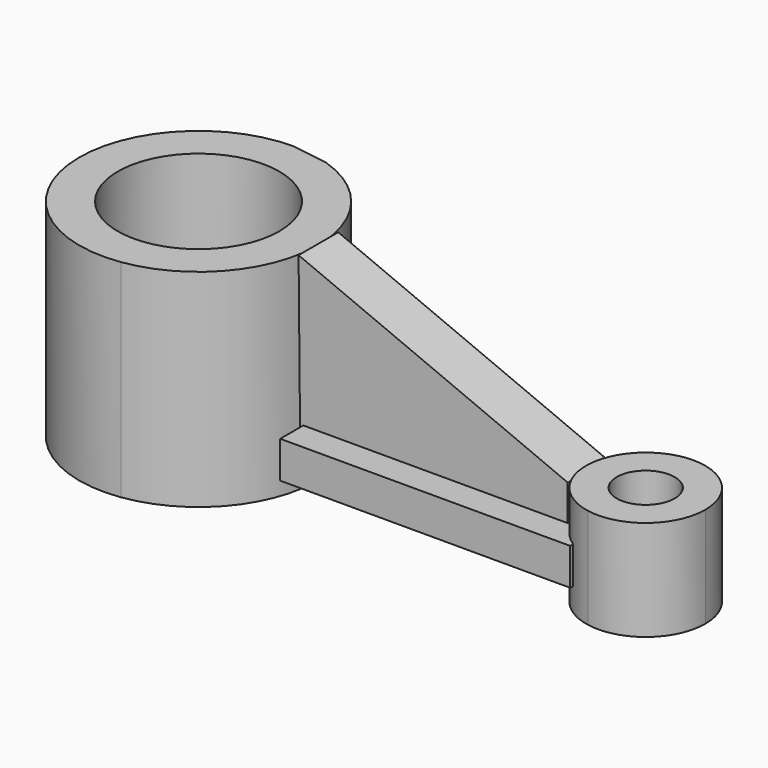
from build123d import *

# Parameters (mm, degrees)
F0_R     = 9.2489930255
F2_DEPTH = 32
F0_R_2   = 25.7680619567
F3_DEPTH = 66
F5_DEPTH = 7.9
F6_W     = 92.4349650741
F6_H     = 11.7601733655
F7_DEPTH = 17.1


# Not quite as in the source:
# - the program builds the solid bodies; features that only make, move or delete a surface that nothing else refers to are left out


with BuildPart() as f2:
    # F0 (on Top) → F2 (new body)
    with BuildSketch(Plane.XY):
        with BuildLine():
            ThreePointArc((133.492457104, 16.7202410111), (128.4908183641, 12.8151071715), (125.053801914, 7.4809363539))
            ThreePointArc((125.053801914, 7.4809363539), (123.5444678368, 0.9778584581), (124.3774057894, -5.6459113026))
            ThreePointArc((124.3774057894, -5.6459113026), (129.9444314059, -14.2444809861), (139.1661912203, -18.7038891017))
            ThreePointArc((139.1661912203, -18.7038891017), (154.7146430032, -14.5749919666), (161.5243238744, 0))
            ThreePointArc((161.5243238744, 0), (152.256160322, 16.3198653036), (133.492457104, 16.7202410111))
        make_face()
        with Locations((142.5218075093, 0)):
            Circle(F0_R, mode=Mode.SUBTRACT)
    extrude(amount=F2_DEPTH)

    # F4 (on Front) → F5 (join, symmetric)
    with BuildSketch(Plane.XZ):
        Polygon((123.9959970117, 30.6361690164), (38.2147207856, 66.5446072817), (38.7846939266, 7.2671840899), (123.9959970117, 6.4122211188), align=None)
    extrude(amount=F5_DEPTH, both=True)

    # F6 (on Front) → F7 (join, symmetric)
    with BuildSketch(Plane.XZ):
        with Locations((85.9421528876, 13.3774159476)):
            Rectangle(F6_W, F6_H)
    extrude(amount=F7_DEPTH, both=True)


with BuildPart() as f3:
    # F0 (on Top) → F3 (new body)
    with BuildSketch(Plane.XY):
        with BuildLine():
            ThreePointArc((37.5782341996, -5.6459113026), (37.8944118544, -2.8308214721), (38, 0))
            ThreePointArc((38, 0), (37.8136303979, 3.7589035813), (37.2563496772, 7.4809363539))
            ThreePointArc((37.2563496772, 7.4809363539), (28.4076518531, 25.2389642457), (11.8147801023, 36.1166301187))
            Line((11.8147801023, 36.1166301187), (0, 38))
            ThreePointArc((0, 38), (-37.9063529214, -2.666159823), (5.3191786945, -37.6258732525))
            ThreePointArc((5.3191786945, -37.6258732525), (26.7530652418, -26.9865429458), (37.5782341996, -5.6459113026))
        make_face()
        Circle(F0_R_2, mode=Mode.SUBTRACT)
    extrude(amount=F3_DEPTH)


solid = Compound([f2.part, f3.part])
